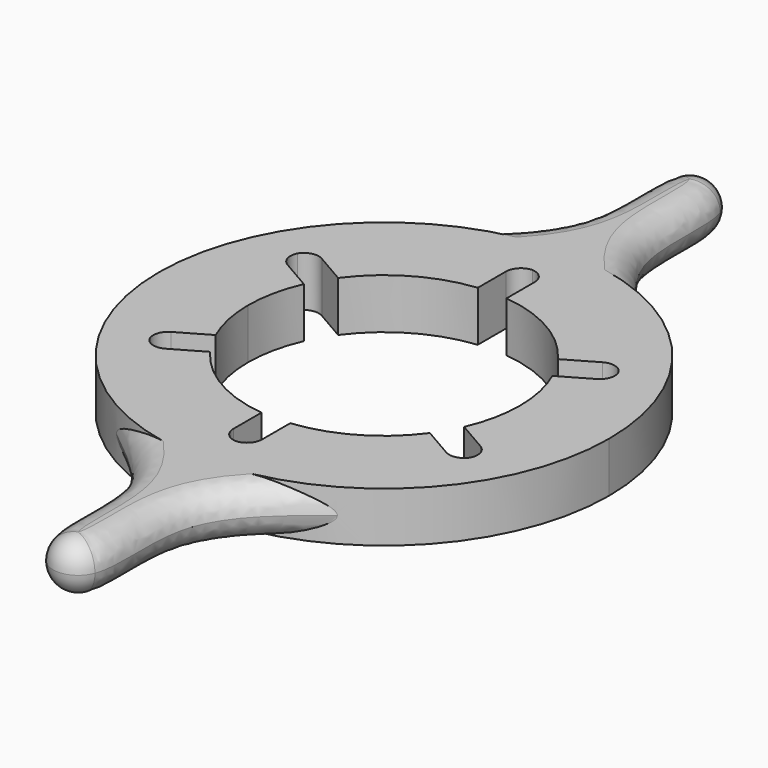
from build123d import *

# Parameters (mm, degrees)
F1_DEPTH    = 10.16
F2_T1_DEPTH = 10.16
F3_R        = 5.0799


# Not quite as in the source:
# - a fillet or chamfer that OpenCascade refuses, or shapes differently, is made with other operations: its cross-section is extruded or revolved along the edge and cut away or added
# - a fillet or chamfer is up to 0.001 mm smaller than in the source, because OpenCascade refuses the exact size


with BuildPart() as f1:
    # F0 (on Top) → F1 (new body)
    with BuildSketch(Plane.XY):
        with BuildLine():
            ThreePointArc((25.1343219542, 11.1586674789), (26.9020803446, 5.7033387704), (27.5, 0))
            Line((27.5, 0), (45.5622851679, 0))
            ThreePointArc((45.5622851679, 0), (39.3272729055, 23.00624775), (22.3287079413, 39.7158737962))
            ThreePointArc((22.3287079413, 39.7158737962), (11.5407075634, 44.0764551508), (0, 45.5622851679))
            Line((0, 45.5622851679), (0, 37.5))
            Line((0, 37.5), (2.903471468, 37.5))
            Line((2.903471468, 37.5), (2.903471468, 27.3462950586))
            ThreePointArc((2.903471468, 27.3462950586), (13.75, 23.8156986041), (22.2308504862, 16.1876275798))
            Line((22.2308504862, 16.1876275798), (31.0242169079, 21.2644800505))
            Line((31.0242169079, 21.2644800505), (33.9276883759, 16.2355199495))
            Line((33.9276883759, 16.2355199495), (25.1343219542, 11.1586674789))
        make_face()
        with BuildLine():
            Line((-45.5622851679, 0), (-27.5, 0))
            ThreePointArc((-27.5, 0), (-26.9020803446, 5.7033387704), (-25.1343219542, 11.1586674789))
            Line((-25.1343219542, 11.1586674789), (-33.9276883759, 16.2355199495))
            Line((-33.9276883759, 16.2355199495), (-31.0242169079, 21.2644800505))
            Line((-31.0242169079, 21.2644800505), (-22.2308504862, 16.1876275798))
            ThreePointArc((-22.2308504862, 16.1876275798), (-13.75, 23.8156986041), (-2.903471468, 27.3462950586))
            Line((-2.903471468, 27.3462950586), (-2.903471468, 37.5))
            Line((-2.903471468, 37.5), (0, 37.5))
            Line((0, 37.5), (0, 45.5622851679))
            ThreePointArc((0, 45.5622851679), (-11.5407075634, 44.0764551508), (-22.3287079413, 39.7158737962))
            ThreePointArc((-22.3287079413, 39.7158737962), (-39.3272729055, 23.00624775), (-45.5622851679, 0))
        make_face()
        with BuildLine():
            Line((45.5622851679, 0), (27.5, 0))
            ThreePointArc((27.5, 0), (26.9020803446, -5.7033387704), (25.1343219542, -11.1586674789))
            Line((25.1343219542, -11.1586674789), (33.9276883759, -16.2355199495))
            Line((33.9276883759, -16.2355199495), (31.0242169079, -21.2644800505))
            Line((31.0242169079, -21.2644800505), (22.2308504862, -16.1876275798))
            ThreePointArc((22.2308504862, -16.1876275798), (13.75, -23.8156986041), (2.903471468, -27.3462950586))
            Line((2.903471468, -27.3462950586), (2.903471468, -37.5))
            Line((2.903471468, -37.5), (0, -37.5))
            Line((0, -37.5), (0, -45.5622851679))
            ThreePointArc((0, -45.5622851679), (11.5407075634, -44.0764551508), (22.3287079413, -39.7158737962))
            ThreePointArc((22.3287079413, -39.7158737962), (39.3272729055, -23.00624775), (45.5622851679, 0))
        make_face()
        with BuildLine():
            ThreePointArc((-25.1343219542, -11.1586674789), (-26.9020803446, -5.7033387704), (-27.5, 0))
            Line((-27.5, 0), (-45.5622851679, 0))
            ThreePointArc((-45.5622851679, 0), (-39.3272729055, -23.00624775), (-22.3287079413, -39.7158737962))
            ThreePointArc((-22.3287079413, -39.7158737962), (-11.5407075634, -44.0764551508), (0, -45.5622851679))
            Line((0, -45.5622851679), (0, -37.5))
            Line((0, -37.5), (-2.903471468, -37.5))
            Line((-2.903471468, -37.5), (-2.903471468, -27.3462950586))
            ThreePointArc((-2.903471468, -27.3462950586), (-13.75, -23.8156986041), (-22.2308504862, -16.1876275798))
            Line((-22.2308504862, -16.1876275798), (-31.0242169079, -21.2644800505))
            Line((-31.0242169079, -21.2644800505), (-33.9276883759, -16.2355199495))
            Line((-33.9276883759, -16.2355199495), (-25.1343219542, -11.1586674789))
        make_face()
        with BuildLine():
            ThreePointArc((-22.3287079413, 39.7158737962), (-11.5407075634, 44.0764551508), (0, 45.5622851679))
            Line((0, 45.5622851679), (0, 84.7600996494))
            add(Edge.make_bspline(
                [(-22.3287079413, 39.7158737962), (-15.6217203488, 45.032214178), (-2.6692040012, 55.2647099046), (-7.4863809829, 78.7666979989), (-2.0884758165, 83.0876040959), (0, 84.7600996494)],
                knots=[0, 0, 0, 0, 0.3975921644, 0.7669085627, 1, 1, 1, 1], degree=3))
        make_face()
        with BuildLine():
            ThreePointArc((0, 45.5622851679), (11.5407075634, 44.0764551508), (22.3287079413, 39.7158737962))
            add(Edge.make_bspline(
                [(22.3287079413, 39.7158737962), (15.6217203488, 45.032214178), (2.6692040012, 55.2647099046), (7.4863809829, 78.7666979989), (2.0884758165, 83.0876040959), (0, 84.7600996494)],
                knots=[0, 0, 0, 0, 0.3975921644, 0.7669085627, 1, 1, 1, 1], degree=3))
            Line((0, 84.7600996494), (0, 45.5622851679))
        make_face()
        with BuildLine():
            Line((0, -84.7600996494), (0, -45.5622851679))
            ThreePointArc((0, -45.5622851679), (-11.5407075634, -44.0764551508), (-22.3287079413, -39.7158737962))
            add(Edge.make_bspline(
                [(-22.3287079413, -39.7158737962), (-15.6217203488, -45.032214178), (-2.6692040012, -55.2647099046), (-7.4863809829, -78.7666979989), (-2.0884758165, -83.0876040959), (0, -84.7600996494)],
                knots=[0, 0, 0, 0, 0.3975921644, 0.7669085627, 1, 1, 1, 1], degree=3))
        make_face()
        with BuildLine():
            add(Edge.make_bspline(
                [(22.3287079413, -39.7158737962), (15.6217203488, -45.032214178), (2.6692040012, -55.2647099046), (7.4863809829, -78.7666979989), (2.0884758165, -83.0876040959), (0, -84.7600996494)],
                knots=[0, 0, 0, 0, 0.3975921644, 0.7669085627, 1, 1, 1, 1], degree=3))
            ThreePointArc((22.3287079413, -39.7158737962), (11.5407075634, -44.0764551508), (0, -45.5622851679))
            Line((0, -45.5622851679), (0, -84.7600996494))
        make_face()
    extrude(amount=F1_DEPTH)

    # F2: fillet of radius 3.048 on 12 edges, made by hand

    # F2_s2 → F2_t1 (join)
    with BuildSketch(Plane.XY):
        with BuildLine():
            ThreePointArc((-32.5482169079, 18.6248346197), (-30.6974519266, 20.0449765383), (-28.3845714772, 19.7404800505))
            Line((-28.3845714772, 19.7404800505), (-31.0242169079, 21.2644800505))
            Line((-31.0242169079, 21.2644800505), (-32.5482169079, 18.6248346197))
        make_face()
        with BuildLine():
            ThreePointArc((-31.2880429452, 14.7115199495), (-32.7081848637, 16.5622849308), (-32.4036883759, 18.8751653803))
            Line((-32.4036883759, 18.8751653803), (-33.9276883759, 16.2355199495))
            Line((-33.9276883759, 16.2355199495), (-31.2880429452, 14.7115199495))
        make_face()
        with BuildLine():
            ThreePointArc((-2.903471468, 34.452), (-2.0107329371, 36.6072614691), (0.144528532, 37.5))
            Line((0.144528532, 37.5), (-2.903471468, 37.5))
            Line((-2.903471468, 37.5), (-2.903471468, 34.452))
        make_face()
        with BuildLine():
            ThreePointArc((-0.144528532, 37.5), (2.0107329371, 36.6072614691), (2.903471468, 34.452))
            Line((2.903471468, 34.452), (2.903471468, 37.5))
            Line((2.903471468, 37.5), (-0.144528532, 37.5))
        make_face()
        with BuildLine():
            ThreePointArc((28.3845714772, 19.7404800505), (30.6974519266, 20.0449765383), (32.5482169079, 18.6248346197))
            Line((32.5482169079, 18.6248346197), (31.0242169079, 21.2644800505))
            Line((31.0242169079, 21.2644800505), (28.3845714772, 19.7404800505))
        make_face()
        with BuildLine():
            ThreePointArc((32.4036883759, 18.8751653803), (32.7081848637, 16.5622849308), (31.2880429452, 14.7115199495))
            Line((31.2880429452, 14.7115199495), (33.9276883759, 16.2355199495))
            Line((33.9276883759, 16.2355199495), (32.4036883759, 18.8751653803))
        make_face()
        with BuildLine():
            ThreePointArc((-32.4036883759, -18.8751653803), (-32.7081848637, -16.5622849308), (-31.2880429452, -14.7115199495))
            Line((-31.2880429452, -14.7115199495), (-33.9276883759, -16.2355199495))
            Line((-33.9276883759, -16.2355199495), (-32.4036883759, -18.8751653803))
        make_face()
        with BuildLine():
            ThreePointArc((-28.3845714772, -19.7404800505), (-30.6974519266, -20.0449765383), (-32.5482169079, -18.6248346197))
            Line((-32.5482169079, -18.6248346197), (-31.0242169079, -21.2644800505))
            Line((-31.0242169079, -21.2644800505), (-28.3845714772, -19.7404800505))
        make_face()
        with BuildLine():
            ThreePointArc((32.5482169079, -18.6248346197), (30.6974519266, -20.0449765383), (28.3845714772, -19.7404800505))
            Line((28.3845714772, -19.7404800505), (31.0242169079, -21.2644800505))
            Line((31.0242169079, -21.2644800505), (32.5482169079, -18.6248346197))
        make_face()
        with BuildLine():
            ThreePointArc((31.2880429452, -14.7115199495), (32.7081848637, -16.5622849308), (32.4036883759, -18.8751653803))
            Line((32.4036883759, -18.8751653803), (33.9276883759, -16.2355199495))
            Line((33.9276883759, -16.2355199495), (31.2880429452, -14.7115199495))
        make_face()
        with BuildLine():
            ThreePointArc((2.903471468, -34.452), (2.0107329371, -36.6072614691), (-0.144528532, -37.5))
            Line((-0.144528532, -37.5), (2.903471468, -37.5))
            Line((2.903471468, -37.5), (2.903471468, -34.452))
        make_face()
        with BuildLine():
            ThreePointArc((0.144528532, -37.5), (-2.0107329371, -36.6072614691), (-2.903471468, -34.452))
            Line((-2.903471468, -34.452), (-2.903471468, -37.5))
            Line((-2.903471468, -37.5), (0.144528532, -37.5))
        make_face()
    extrude(amount=F2_T1_DEPTH)

    # F3 (radius 5.08 in the source; OpenCascade refuses exactly that, so slightly less here)
    f3_edges = [f1.edges().sort_by_distance(p)[0] for p in [
        (6.10989, -60.06232, 10.16),
        (6.10989, -60.06232, 0),
        (-6.10989, -60.06232, 10.16),
        (-6.10989, -60.06232, 0),
        (0, -84.7601, 5.08),
        (6.10989, 60.06232, 10.16),
        (-6.10989, 60.06232, 10.16),
        (0, 84.7601, 5.08),
        (6.10989, 60.06232, 0),
        (-6.10989, 60.06232, 0),
    ]]
    fillet(f3_edges, radius=F3_R)


solid = f1.part
